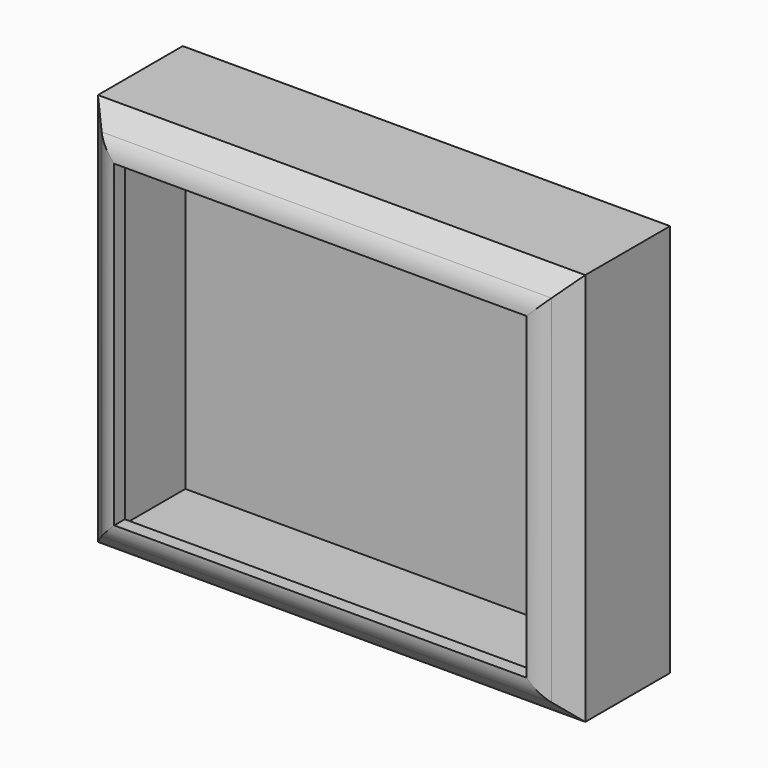
from build123d import *

# Parameters (mm, degrees)
F0_W     = 93.4118106961
F0_H     = 75.4010342062
F1_DEPTH = 25.4
F2_SIZE  = 5.08
F3_R     = 5.08
F4_T     = -2.54


# Not quite as in the source:
# - a shell that OpenCascade refuses in one call is made with other operations: the cavity is built on its own and cut out


with BuildPart() as f1:
    # F0 (on Front) → F1 (new body)
    with BuildSketch(Plane.XZ):
        with Locations((0.4579015076, -3.3579412848)):
            Rectangle(F0_W, F0_H)
    extrude(amount=F1_DEPTH)

    # F2
    f2_edges = [f1.edges().sort_by_distance(p)[0] for p in [
        (0.457902, -25.4, 34.342576),
        (-46.248004, -25.4, -3.357941),
        (0.457902, -25.4, -41.058458),
        (47.163807, -25.4, -3.357941),
    ]]
    chamfer(f2_edges, length=F2_SIZE)

    # F3
    f3_edges = [f1.edges().sort_by_distance(p)[0] for p in [
        (0.457902, -25.4, 29.262576),
        (42.083807, -25.4, -3.357941),
        (-41.168004, -25.4, -3.357941),
        (0.457902, -25.4, -35.978458),
    ]]
    fillet(f3_edges, radius=F3_R)

    # F4: a shell. OpenCascade refuses it in one call, so the cavity is built on its own and cut out:
    # the body offset inwards by the wall thickness, plus a prism from it out through each open face.
    f4_core = offset(f1.part, amount=F4_T, mode=Mode.PRIVATE)
    f4_exits = [f4_core.faces().sort_by_distance(p)[0] for p in [
        (0.457902, -22.86, -3.357941),
    ]]
    add(f4_core, mode=Mode.SUBTRACT)
    extrude(f4_exits, amount=-F4_T, mode=Mode.SUBTRACT)


solid = f1.part
